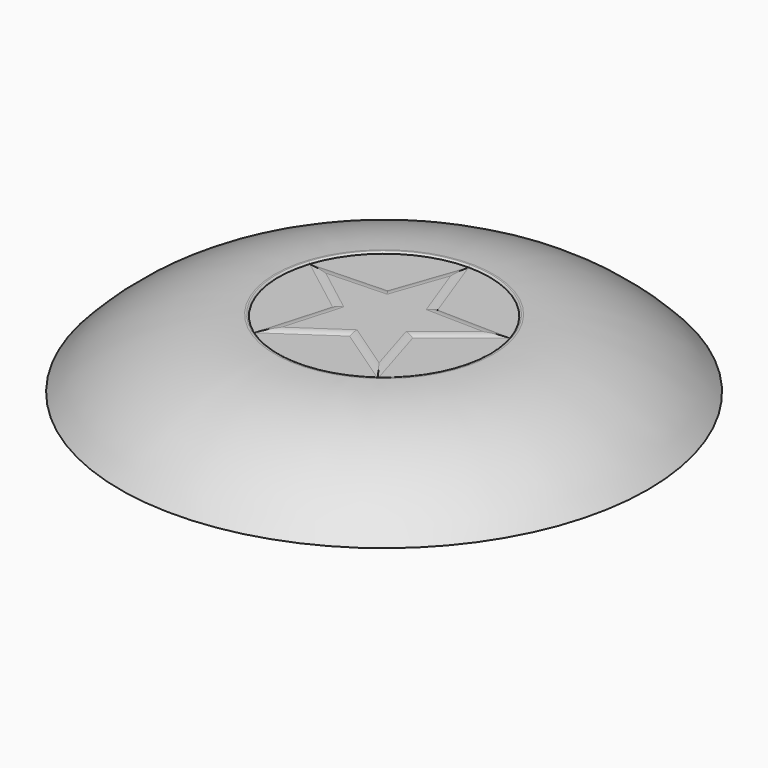
from build123d import *

# Parameters (mm, degrees)
F1_DEPTH      = 19.5
F2_DEPTH      = 19
F3_T4_DEPTH   = 32.6000135718
F3_T9_DEPTH   = 31.9798965953
F3_T14_DEPTH  = 32.5094005548
F3_T19_DEPTH  = 32.0663833981
F3_T24_DEPTH  = 32.41943719
F3_T29_DEPTH  = 32.1535963091
F3_T34_DEPTH  = 32.3301385521
F3_T39_DEPTH  = 32.241519827
F3_T44_DEPTH  = 32.241519827
F3_T49_DEPTH  = 31.8941515
F3_T55_DEPTH  = 32.6000135718
F3_T59_DEPTH  = 31.8941515
F3_T66_DEPTH  = 32.5094005548
F3_T70_DEPTH  = 31.9798965953
F3_T77_DEPTH  = 32.41943719
F3_T81_DEPTH  = 32.0663833981
F3_T88_DEPTH  = 32.3301385521
F3_T92_DEPTH  = 32.1535963091
F3_T99_DEPTH  = 32.241519827
F3_T103_DEPTH = 32.241519827
F0_R          = 45
F4_DEPTH      = 19.5
F5_R          = 0.49999
F0_R_2        = 75
F0_R_3        = 60
F6_DEPTH      = 19.5


# Not quite as in the source:
# - a fillet or chamfer that OpenCascade refuses, or shapes differently, is made with other operations: its cross-section is extruded or revolved along the edge and cut away or added
# - a fillet or chamfer is up to 0.001 mm smaller than in the source, because OpenCascade refuses the exact size
# - the program builds the solid bodies; features that only make, move or delete a surface that nothing else refers to are left out


with BuildPart() as f1:
    # F0 (on Top) → F1 (new body)
    with BuildSketch(Plane.XY):
        Polygon((11.5056481768, -4.1877134623), (28.5316954889, 9.2705098312), (7.4537084477, 9.7138619707), (0, 30), (-7.0229014607, 10.0297427227), (-28.5316954889, 9.2705098312), (-11.6773628448, -3.6818583623), (-17.6335575688, -24.2705098312), (0, -12.2440550476), (17.6335575688, -24.2705098312), align=None)
    extrude(amount=F1_DEPTH)

    # F0 (on Top) → F2 (join)
    with BuildSketch(Plane.XY):
        with BuildLine():
            Line((7.4537084477, 9.7138619707), (28.5316954889, 9.2705098312))
            ThreePointArc((28.5316954889, 9.2705098312), (17.6335575688, 24.2705098312), (0, 30))
            Line((0, 30), (7.4537084477, 9.7138619707))
        make_face()
        with BuildLine():
            Line((-7.0229014607, 10.0297427227), (0, 30))
            ThreePointArc((0, 30), (-17.6335575688, 24.2705098312), (-28.5316954889, 9.2705098312))
            Line((-28.5316954889, 9.2705098312), (-7.0229014607, 10.0297427227))
        make_face()
        with BuildLine():
            ThreePointArc((-28.5316954889, 9.2705098312), (-28.5316954889, -9.2705098312), (-17.6335575688, -24.2705098312))
            Line((-17.6335575688, -24.2705098312), (-11.6773628448, -3.6818583623))
            Line((-11.6773628448, -3.6818583623), (-28.5316954889, 9.2705098312))
        make_face()
        with BuildLine():
            ThreePointArc((-17.6335575688, -24.2705098312), (0, -30), (17.6335575688, -24.2705098312))
            Line((17.6335575688, -24.2705098312), (0, -12.2440550476))
            Line((0, -12.2440550476), (-17.6335575688, -24.2705098312))
        make_face()
        with BuildLine():
            ThreePointArc((17.6335575688, -24.2705098312), (26.7301957257, -13.6197149922), (30, 0))
            ThreePointArc((30, 0), (29.6306502179, 4.6930339512), (28.5316954889, 9.2705098312))
            Line((28.5316954889, 9.2705098312), (11.5056481768, -4.1877134623))
            Line((11.5056481768, -4.1877134623), (17.6335575688, -24.2705098312))
        make_face()
    extrude(amount=F2_DEPTH)

    # F3: fillet of radius 5 on 10 edges, made by hand


with BuildPart() as f3_tool2:
    # F3_s3 → F3_t4 (new body)
    with BuildSketch(Plane(origin=(0.7694568459, 0.6082164496, 0), x_dir=(0, 0, 1), z_dir=(0.7845104695, 0.6201155724, 0))):
        with BuildLine():
            ThreePointArc((19, 10.42013666), (19.3733971724, 9.3587211769), (19.5, 8.2406871882))
            Line((19.5, 8.2406871882), (19.5, 10.42013666))
            Line((19.5, 10.42013666), (19, 10.42013666))
        make_face()
    extrude(amount=F3_T4_DEPTH)

    split(bisect_by=Plane(origin=(9.3566812143, 2.8550254475, 0), x_dir=(0, 0, 1), z_dir=(0.9564646404, 0.2918482339, 0)), keep=Keep.TOP)


with BuildPart() as f1_1:
    add(f1.part)

    # F3_t1: cut F3_tool2
    add(f3_tool2.part, mode=Mode.SUBTRACT)


with BuildPart() as f3_tool7:
    # F3_s8 → F3_t9 (new body)
    with BuildSketch(Plane(origin=(33.771588035, -0.7103479939, 0), x_dir=(0, 0, 1), z_dir=(-0.999778861, 0.0210292423, 0))):
        with BuildLine():
            ThreePointArc((19.5, 7.6890102267), (19.3733971724, 8.8070442154), (19, 9.8684596985))
            Line((19, 9.8684596985), (19.5, 9.8684596985))
            Line((19.5, 9.8684596985), (19.5, 7.6890102267))
        make_face()
    extrude(amount=F3_T9_DEPTH)

    split(bisect_by=Plane(origin=(9.7117379965, 3.5683708472, 0), x_dir=(0, 0, 1), z_dir=(0.9386449303, 0.3448850459, 0)), keep=Keep.TOP)


with BuildPart() as f1_2:
    add(f1_1.part)

    # F3_t6: cut F3_tool7
    add(f3_tool7.part, mode=Mode.SUBTRACT)


with BuildPart() as f3_tool12:
    # F3_s13 → F3_t14 (new body)
    with BuildSketch(Plane(origin=(-0.3788807209, 1.03116813, 0), x_dir=(0, 0, 1), z_dir=(-0.3448850459, 0.9386449303, 0))):
        with BuildLine():
            ThreePointArc((19, 10.3465513779), (19.3733971724, 9.2851358949), (19.5, 8.1671019062))
            Line((19.5, 8.1671019062), (19.5, 10.3465513779))
            Line((19.5, 10.3465513779), (19, 10.3465513779))
        make_face()
    extrude(amount=F3_T14_DEPTH)

    split(bisect_by=Plane(origin=(0.2075262303, 9.8662773975, 0), x_dir=(0, 0, 1), z_dir=(0.0210292423, 0.999778861, 0)), keep=Keep.TOP)


with BuildPart() as f1_3:
    add(f1_2.part)

    # F3_t11: cut F3_tool12
    add(f3_tool12.part, mode=Mode.SUBTRACT)


with BuildPart() as f3_tool17:
    # F3_s18 → F3_t19 (new body)
    with BuildSketch(Plane(origin=(11.1965023398, 31.8382699206, 0), x_dir=(0, 0, 1), z_dir=(-0.3317519169, -0.9433666655, 0))):
        with BuildLine():
            ThreePointArc((19, 9.9525575078), (19.3733971724, 8.8911420248), (19.5, 7.773108036))
            Line((19.5, 7.773108036), (19.5, 9.9525575078))
            Line((19.5, 9.9525575078), (19, 9.9525575078))
        make_face()
    extrude(amount=F3_T19_DEPTH)

    split(bisect_by=Plane(origin=(-0.3623361388, 10.264852151, 0), x_dir=(0, 0, 1), z_dir=(-0.0352767491, 0.9993775818, 0)), keep=Keep.TOP)


with BuildPart() as f1_4:
    add(f1_3.part)

    # F3_t16: cut F3_tool17
    add(f3_tool17.part, mode=Mode.SUBTRACT)


with BuildPart() as f3_tool22:
    # F3_s23 → F3_t24 (new body)
    with BuildSketch(Plane(origin=(-1.2153329651, -0.0428996977, 0), x_dir=(0, 0, 1), z_dir=(-0.9993775818, -0.0352767491, 0))):
        with BuildLine():
            ThreePointArc((19, 10.2712451611), (19.3733971724, 9.209829678), (19.5, 8.0917956893))
            Line((19.5, 8.0917956893), (19.5, 10.2712451611))
            Line((19.5, 10.2712451611), (19, 10.2712451611))
        make_face()
    extrude(amount=F3_T24_DEPTH)

    split(bisect_by=Plane(origin=(-9.3889109895, 3.3017800315, 0), x_dir=(0, 0, 1), z_dir=(-0.9433666655, 0.3317519169, 0)), keep=Keep.TOP)


with BuildPart() as f1_5:
    add(f1_4.part)

    # F3_t21: cut F3_tool22
    add(f3_tool22.part, mode=Mode.SUBTRACT)


with BuildPart() as f3_tool27:
    # F3_s28 → F3_t29 (new body)
    with BuildSketch(Plane(origin=(-26.7372924148, 20.5473134516, 0), x_dir=(0, 0, 1), z_dir=(0.7929081652, -0.6093411537, 0))):
        with BuildLine():
            ThreePointArc((19, 10.0348733068), (19.3733971724, 8.9734578238), (19.5, 7.855423835))
            Line((19.5, 7.855423835), (19.5, 10.0348733068))
            Line((19.5, 10.0348733068), (19, 10.0348733068))
        make_face()
    extrude(amount=F3_T29_DEPTH)

    split(bisect_by=Plane(origin=(-9.792656229, 2.832966863, 0), x_dir=(0, 0, 1), z_dir=(-0.9606100868, 0.2778997323, 0)), keep=Keep.TOP)


with BuildPart() as f1_6:
    add(f1_5.part)

    # F3_t26: cut F3_tool27
    add(f3_tool27.part, mode=Mode.SUBTRACT)


with BuildPart() as f3_tool32:
    # F3_s33 → F3_t34 (new body)
    with BuildSketch(Plane(origin=(-0.3705355542, -1.2808223597, 0), x_dir=(0, 0, 1), z_dir=(-0.2778997323, -0.9606100868, 0))):
        with BuildLine():
            ThreePointArc((19, 10.1942050826), (19.3733971724, 9.1327895996), (19.5, 8.0147556108))
            Line((19.5, 8.0147556108), (19.5, 10.1942050826))
            Line((19.5, 10.1942050826), (19, 10.1942050826))
        make_face()
    extrude(amount=F3_T34_DEPTH)

    split(bisect_by=Plane(origin=(-6.1146612783, -7.9567329812, 0), x_dir=(0, 0, 1), z_dir=(-0.6093411537, -0.7929081652, 0)), keep=Keep.TOP)


with BuildPart() as f1_7:
    add(f1_6.part)

    # F3_t31: cut F3_tool32
    add(f3_tool32.part, mode=Mode.SUBTRACT)


with BuildPart() as f3_tool37:
    # F3_s38 → F3_t39 (new body)
    with BuildSketch(Plane(origin=(-27.8344788416, -18.9836962796, 0), x_dir=(0, 0, 1), z_dir=(0.8261493848, 0.563451146, 0))):
        with BuildLine():
            ThreePointArc((19, 10.1154185452), (19.3733971724, 9.0540030622), (19.5, 7.9359690734))
            Line((19.5, 7.9359690734), (19.5, 10.1154185452))
            Line((19.5, 10.1154185452), (19, 10.1154185452))
        make_face()
    extrude(amount=F3_T39_DEPTH)

    split(bisect_by=Plane(origin=(-5.699544172, -8.3568468082, 0), x_dir=(0, 0, 1), z_dir=(-0.563451146, -0.8261493848, 0)), keep=Keep.TOP)


with BuildPart() as f1_8:
    add(f1_7.part)

    # F3_t36: cut F3_tool37
    add(f3_tool37.part, mode=Mode.SUBTRACT)


with BuildPart() as f3_tool42:
    # F3_s43 → F3_t44 (new body)
    with BuildSketch(Plane(origin=(1.1981670712, -0.8171749829, 0), x_dir=(0, 0, 1), z_dir=(0.8261493848, -0.563451146, 0))):
        with BuildLine():
            ThreePointArc((19, 10.1154185452), (19.3733971724, 9.0540030622), (19.5, 7.9359690734))
            Line((19.5, 7.9359690734), (19.5, 10.1154185452))
            Line((19.5, 10.1154185452), (19, 10.1154185452))
        make_face()
    extrude(amount=F3_T44_DEPTH)

    split(bisect_by=Plane(origin=(5.699544172, -8.3568468082, 0), x_dir=(0, 0, 1), z_dir=(0.563451146, -0.8261493848, 0)), keep=Keep.TOP)


with BuildPart() as f1_9:
    add(f1_8.part)

    # F3_t41: cut F3_tool42
    add(f3_tool42.part, mode=Mode.SUBTRACT)


with BuildPart() as f3_tool47:
    # F3_s48 → F3_t49 (new body)
    with BuildSketch(Plane(origin=(9.8670475528, -32.336951167, 0), x_dir=(0, 0, 1), z_dir=(-0.2918482339, 0.9564646404, 0))):
        with BuildLine():
            ThreePointArc((19, 9.7825688677), (19.3733971724, 8.7211533847), (19.5, 7.603119396))
            Line((19.5, 7.603119396), (19.5, 9.7825688677))
            Line((19.5, 9.7825688677), (19, 9.7825688677))
        make_face()
    extrude(amount=F3_T49_DEPTH)

    split(bisect_by=Plane(origin=(6.4616890097, -8.1747063038, 0), x_dir=(0, 0, 1), z_dir=(0.6201155724, -0.7845104695, 0)), keep=Keep.TOP)


with BuildPart() as f1_10:
    add(f1_9.part)

    # F3_t46: cut F3_tool47
    add(f3_tool47.part, mode=Mode.SUBTRACT)


with BuildPart() as f3_tool53:
    # F3_s54 → F3_t55 (new body)
    with BuildSketch(Plane(origin=(0.7694568459, 0.6082164496, 0), x_dir=(0, 0, 1), z_dir=(0.7845104695, 0.6201155724, 0))):
        with BuildLine():
            ThreePointArc((19, 10.42013666), (19.3733971724, 9.3587211769), (19.5, 8.2406871882))
            Line((19.5, 8.2406871882), (19.5, 10.42013666))
            Line((19.5, 10.42013666), (19, 10.42013666))
        make_face()
    extrude(amount=F3_T55_DEPTH)

    split(bisect_by=Plane(origin=(9.3566812143, 2.8550254475, 0), x_dir=(0, 0, 1), z_dir=(-0.9564646404, -0.2918482339, 0)), keep=Keep.TOP)


with BuildPart() as f3_tool57:
    # F3_s58 → F3_t59 (new body)
    with BuildSketch(Plane(origin=(9.8670475528, -32.336951167, 0), x_dir=(0, 0, 1), z_dir=(-0.2918482339, 0.9564646404, 0))):
        with BuildLine():
            ThreePointArc((19, 9.7825688677), (19.3733971724, 8.7211533847), (19.5, 7.603119396))
            Line((19.5, 7.603119396), (19.5, 9.7825688677))
            Line((19.5, 9.7825688677), (19, 9.7825688677))
        make_face()
    extrude(amount=F3_T59_DEPTH)

    split(bisect_by=Plane(origin=(6.4616890097, -8.1747063038, 0), x_dir=(0, 0, 1), z_dir=(-0.6201155724, 0.7845104695, 0)), keep=Keep.TOP)


with BuildPart() as f3_tool53_1:
    add(f3_tool53.part)

    # F3_t61: intersect F3_tool57
    add(f3_tool57.part, mode=Mode.INTERSECT)


with BuildPart() as f1_11:
    add(f1_10.part)

    # F3_t51: cut F3_tool53
    add(f3_tool53_1.part, mode=Mode.SUBTRACT)


with BuildPart() as f3_tool64:
    # F3_s65 → F3_t66 (new body)
    with BuildSketch(Plane(origin=(-0.3788807209, 1.03116813, 0), x_dir=(0, 0, 1), z_dir=(-0.3448850459, 0.9386449303, 0))):
        with BuildLine():
            ThreePointArc((19, 10.3465513779), (19.3733971724, 9.2851358949), (19.5, 8.1671019062))
            Line((19.5, 8.1671019062), (19.5, 10.3465513779))
            Line((19.5, 10.3465513779), (19, 10.3465513779))
        make_face()
    extrude(amount=F3_T66_DEPTH)

    split(bisect_by=Plane(origin=(0.2075262303, 9.8662773975, 0), x_dir=(0, 0, 1), z_dir=(-0.0210292423, -0.999778861, 0)), keep=Keep.TOP)


with BuildPart() as f3_tool68:
    # F3_s69 → F3_t70 (new body)
    with BuildSketch(Plane(origin=(33.771588035, -0.7103479939, 0), x_dir=(0, 0, 1), z_dir=(-0.999778861, 0.0210292423, 0))):
        with BuildLine():
            ThreePointArc((19.5, 7.6890102267), (19.3733971724, 8.8070442154), (19, 9.8684596985))
            Line((19, 9.8684596985), (19.5, 9.8684596985))
            Line((19.5, 9.8684596985), (19.5, 7.6890102267))
        make_face()
    extrude(amount=F3_T70_DEPTH)

    split(bisect_by=Plane(origin=(9.7117379965, 3.5683708472, 0), x_dir=(0, 0, 1), z_dir=(-0.9386449303, -0.3448850459, 0)), keep=Keep.TOP)


with BuildPart() as f3_tool64_1:
    add(f3_tool64.part)

    # F3_t72: intersect F3_tool68
    add(f3_tool68.part, mode=Mode.INTERSECT)


with BuildPart() as f1_12:
    add(f1_11.part)

    # F3_t62: cut F3_tool64
    add(f3_tool64_1.part, mode=Mode.SUBTRACT)


with BuildPart() as f3_tool75:
    # F3_s76 → F3_t77 (new body)
    with BuildSketch(Plane(origin=(-1.2153329651, -0.0428996977, 0), x_dir=(0, 0, 1), z_dir=(-0.9993775818, -0.0352767491, 0))):
        with BuildLine():
            ThreePointArc((19, 10.2712451611), (19.3733971724, 9.209829678), (19.5, 8.0917956893))
            Line((19.5, 8.0917956893), (19.5, 10.2712451611))
            Line((19.5, 10.2712451611), (19, 10.2712451611))
        make_face()
    extrude(amount=F3_T77_DEPTH)

    split(bisect_by=Plane(origin=(-9.3889109895, 3.3017800315, 0), x_dir=(0, 0, 1), z_dir=(0.9433666655, -0.3317519169, 0)), keep=Keep.TOP)


with BuildPart() as f3_tool79:
    # F3_s80 → F3_t81 (new body)
    with BuildSketch(Plane(origin=(11.1965023398, 31.8382699206, 0), x_dir=(0, 0, 1), z_dir=(-0.3317519169, -0.9433666655, 0))):
        with BuildLine():
            ThreePointArc((19, 9.9525575078), (19.3733971724, 8.8911420248), (19.5, 7.773108036))
            Line((19.5, 7.773108036), (19.5, 9.9525575078))
            Line((19.5, 9.9525575078), (19, 9.9525575078))
        make_face()
    extrude(amount=F3_T81_DEPTH)

    split(bisect_by=Plane(origin=(-0.3623361388, 10.264852151, 0), x_dir=(0, 0, 1), z_dir=(0.0352767491, -0.9993775818, 0)), keep=Keep.TOP)


with BuildPart() as f3_tool75_1:
    add(f3_tool75.part)

    # F3_t83: intersect F3_tool79
    add(f3_tool79.part, mode=Mode.INTERSECT)


with BuildPart() as f1_13:
    add(f1_12.part)

    # F3_t73: cut F3_tool75
    add(f3_tool75_1.part, mode=Mode.SUBTRACT)


with BuildPart() as f3_tool86:
    # F3_s87 → F3_t88 (new body)
    with BuildSketch(Plane(origin=(-0.3705355542, -1.2808223597, 0), x_dir=(0, 0, 1), z_dir=(-0.2778997323, -0.9606100868, 0))):
        with BuildLine():
            ThreePointArc((19, 10.1942050826), (19.3733971724, 9.1327895996), (19.5, 8.0147556108))
            Line((19.5, 8.0147556108), (19.5, 10.1942050826))
            Line((19.5, 10.1942050826), (19, 10.1942050826))
        make_face()
    extrude(amount=F3_T88_DEPTH)

    split(bisect_by=Plane(origin=(-6.1146612783, -7.9567329812, 0), x_dir=(0, 0, 1), z_dir=(0.6093411537, 0.7929081652, 0)), keep=Keep.TOP)


with BuildPart() as f3_tool90:
    # F3_s91 → F3_t92 (new body)
    with BuildSketch(Plane(origin=(-26.7372924148, 20.5473134516, 0), x_dir=(0, 0, 1), z_dir=(0.7929081652, -0.6093411537, 0))):
        with BuildLine():
            ThreePointArc((19, 10.0348733068), (19.3733971724, 8.9734578238), (19.5, 7.855423835))
            Line((19.5, 7.855423835), (19.5, 10.0348733068))
            Line((19.5, 10.0348733068), (19, 10.0348733068))
        make_face()
    extrude(amount=F3_T92_DEPTH)

    split(bisect_by=Plane(origin=(-9.792656229, 2.832966863, 0), x_dir=(0, 0, 1), z_dir=(0.9606100868, -0.2778997323, 0)), keep=Keep.TOP)


with BuildPart() as f3_tool86_1:
    add(f3_tool86.part)

    # F3_t94: intersect F3_tool90
    add(f3_tool90.part, mode=Mode.INTERSECT)


with BuildPart() as f1_14:
    add(f1_13.part)

    # F3_t84: cut F3_tool86
    add(f3_tool86_1.part, mode=Mode.SUBTRACT)


with BuildPart() as f3_tool97:
    # F3_s98 → F3_t99 (new body)
    with BuildSketch(Plane(origin=(1.1981670712, -0.8171749829, 0), x_dir=(0, 0, 1), z_dir=(0.8261493848, -0.563451146, 0))):
        with BuildLine():
            ThreePointArc((19, 10.1154185452), (19.3733971724, 9.0540030622), (19.5, 7.9359690734))
            Line((19.5, 7.9359690734), (19.5, 10.1154185452))
            Line((19.5, 10.1154185452), (19, 10.1154185452))
        make_face()
    extrude(amount=F3_T99_DEPTH)

    split(bisect_by=Plane(origin=(5.699544172, -8.3568468082, 0), x_dir=(0, 0, 1), z_dir=(-0.563451146, 0.8261493848, 0)), keep=Keep.TOP)


with BuildPart() as f3_tool101:
    # F3_s102 → F3_t103 (new body)
    with BuildSketch(Plane(origin=(-27.8344788416, -18.9836962796, 0), x_dir=(0, 0, 1), z_dir=(0.8261493848, 0.563451146, 0))):
        with BuildLine():
            ThreePointArc((19, 10.1154185452), (19.3733971724, 9.0540030622), (19.5, 7.9359690734))
            Line((19.5, 7.9359690734), (19.5, 10.1154185452))
            Line((19.5, 10.1154185452), (19, 10.1154185452))
        make_face()
    extrude(amount=F3_T103_DEPTH)

    split(bisect_by=Plane(origin=(-5.699544172, -8.3568468082, 0), x_dir=(0, 0, 1), z_dir=(0.563451146, 0.8261493848, 0)), keep=Keep.TOP)


with BuildPart() as f3_tool97_1:
    add(f3_tool97.part)

    # F3_t105: intersect F3_tool101
    add(f3_tool101.part, mode=Mode.INTERSECT)


with BuildPart() as f1_15:
    add(f1_14.part)

    # F3_t95: cut F3_tool97
    add(f3_tool97_1.part, mode=Mode.SUBTRACT)

    # F0 (on Top) → F4 (join)
    with BuildSketch(Plane.XY):
        Circle(F0_R)
        with BuildLine():
            ThreePointArc((28.5316954889, 9.2705098312), (29.6306502179, 4.6930339512), (30, 0))
            ThreePointArc((30, 0), (26.7301957257, -13.6197149922), (17.6335575688, -24.2705098312))
            ThreePointArc((17.6335575688, -24.2705098312), (0, -30), (-17.6335575688, -24.2705098312))
            ThreePointArc((-17.6335575688, -24.2705098312), (-28.5316954889, -9.2705098312), (-28.5316954889, 9.2705098312))
            ThreePointArc((-28.5316954889, 9.2705098312), (-17.6335575688, 24.2705098312), (0, 30))
            ThreePointArc((0, 30), (17.6335575688, 24.2705098312), (28.5316954889, 9.2705098312))
        make_face(mode=Mode.SUBTRACT)
    extrude(amount=F4_DEPTH)

    # F5 (radius 0.5 in the source; OpenCascade refuses exactly that, so slightly less here)
    f5_edges = [f1_15.edges().sort_by_distance(p)[0] for p in [
        (-17.633558, 24.27051, 19.5),
    ]]
    fillet(f5_edges, radius=F5_R)

    # F0 (on Top) → F6 (join)
    with BuildSketch(Plane.XY):
        Circle(F0_R_2)
        Circle(F0_R_3, mode=Mode.SUBTRACT)
        Circle(F0_R_3)
        Circle(F0_R, mode=Mode.SUBTRACT)
    extrude(amount=F6_DEPTH)

    # F7: fillet of radius 60 on 2 edges, made by hand

    # F7_s1 → F7_t2 (revolve, cut)
    with BuildSketch(Plane.XZ):
        with BuildLine():
            ThreePointArc((30.4980527473, 19.499996247), (54.8111578273, 14.4560946794), (75, 0))
            Line((75, 0), (79.4269472281, 4.049955338))
            ThreePointArc((79.4269472281, 4.049955338), (81, 9.75), (81, 19.5))
            Line((81, 19.5), (75, 25.5))
            ThreePointArc((75, 25.5), (30.49999, 25.5), (30.4748052502, 25.4999512096))
            Line((30.4748052502, 25.4999512096), (30.4980527473, 19.499996247))
        make_face()
    revolve(axis=Axis((0, 0, 19.5), (0, 0, 1)), mode=Mode.SUBTRACT)


solid = f1_15.part
